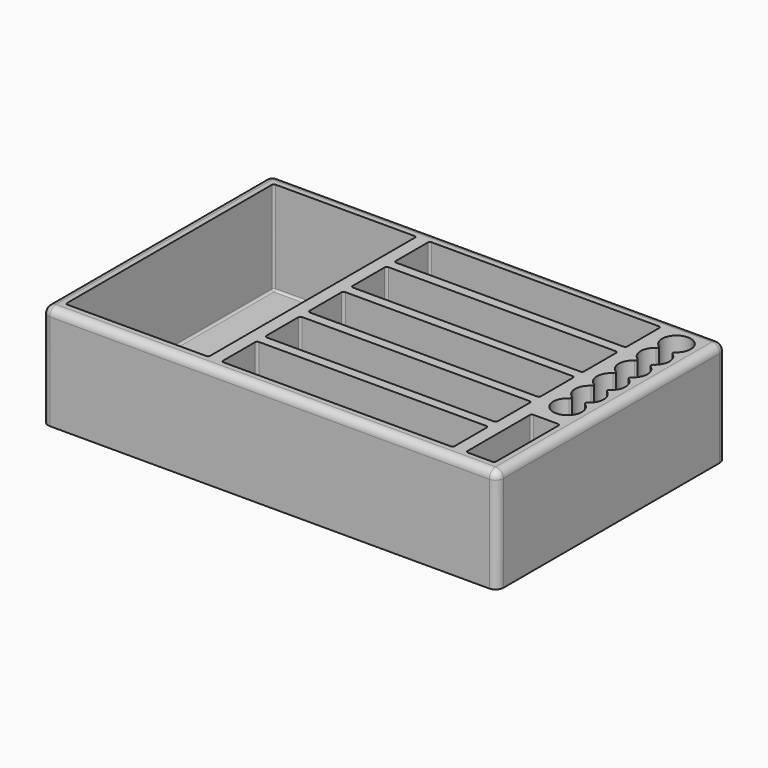
from build123d import *

# Parameters (mm, degrees)
F0_W     = 175
F0_H     = 110
F1_DEPTH = 40
F2_W     = 55
F2_H     = 100
F2_W_2   = 89
F2_H_2   = 17
F2_W_3   = 11
F2_H_3   = 31.5
F3_DEPTH = 36
F4_R     = 0.8068048306
F5_R     = 3


# Not quite as in the source:
# - a feature names something its author has since deleted; it is built from what else it names


with BuildPart() as f1:
    # F0 (on Top) → F1 (new body)
    with BuildSketch(Plane.XY):
        Rectangle(F0_W, F0_H)
    extrude(amount=F1_DEPTH)

    # F2 (on face) → F3 (cut)
    with BuildSketch(Plane.XY.offset(40)):
        with Locations((-55, 0)):
            Rectangle(F2_W, F2_H)
        with Locations((22, 41.5)):
            Rectangle(F2_W_2, F2_H_2)
        with Locations((22, 20.75)):
            Rectangle(F2_W_2, F2_H_2)
        with BuildLine():
            ThreePointArc((78.6393596311, 28.75), (81.4309410948, 30.7416628452), (82.5, 34))
            ThreePointArc((82.5, 34), (81.5093705676, 37.1489009327), (78.8943356059, 39.163476795))
            ThreePointArc((78.8943356059, 39.163476795), (77, 38.8269535899), (75.1056643941, 39.163476795))
            ThreePointArc((75.1056643941, 39.163476795), (71.5016479517, 33.8653717964), (75.3606403689, 28.75))
            ThreePointArc((75.3606403689, 28.75), (77, 29), (78.6393596311, 28.75))
        make_face()
        with BuildLine():
            ThreePointArc((75.1056643941, 39.163476795), (77, 38.8269535899), (78.8943356059, 39.163476795))
            ThreePointArc((78.8943356059, 39.163476795), (77, 39.5), (75.1056643941, 39.163476795))
        make_face()
        with BuildLine():
            ThreePointArc((75.1056643941, 39.163476795), (77, 39.5), (78.8943356059, 39.163476795))
            ThreePointArc((78.8943356059, 39.163476795), (81.5093705676, 41.1780526573), (82.5, 44.3269535899))
            ThreePointArc((82.5, 44.3269535899), (73.8510990673, 48.8363241576), (75.1056643941, 39.163476795))
        make_face()
        with BuildLine():
            ThreePointArc((82.5, 23.5), (81.4309410948, 26.7583371548), (78.6393596311, 28.75))
            ThreePointArc((78.6393596311, 28.75), (77, 28.5), (75.3606403689, 28.75))
            ThreePointArc((75.3606403689, 28.75), (71.5, 23.5), (75.3606403689, 18.25))
            ThreePointArc((75.3606403689, 18.25), (77, 18.5), (78.6393596311, 18.25))
            ThreePointArc((78.6393596311, 18.25), (81.4309410948, 20.2416628452), (82.5, 23.5))
        make_face()
        with BuildLine():
            ThreePointArc((75.3606403689, 28.75), (77, 28.5), (78.6393596311, 28.75))
            ThreePointArc((78.6393596311, 28.75), (77, 29), (75.3606403689, 28.75))
        make_face()
        with BuildLine():
            ThreePointArc((78.6393596311, 18.25), (77, 18.5), (75.3606403689, 18.25))
            ThreePointArc((75.3606403689, 18.25), (77, 18), (78.6393596311, 18.25))
        make_face()
        with BuildLine():
            ThreePointArc((78.6393596311, 18.25), (77, 18), (75.3606403689, 18.25))
            ThreePointArc((75.3606403689, 18.25), (71.5, 13), (75.3606403689, 7.75))
            ThreePointArc((75.3606403689, 7.75), (77, 8), (78.6393596311, 7.75))
            ThreePointArc((78.6393596311, 7.75), (81.4309410948, 9.7416628452), (82.5, 13))
            ThreePointArc((82.5, 13), (81.4309410948, 16.2583371548), (78.6393596311, 18.25))
        make_face()
        with BuildLine():
            ThreePointArc((78.6393596311, 7.75), (77, 8), (75.3606403689, 7.75))
            ThreePointArc((75.3606403689, 7.75), (77, 7.5), (78.6393596311, 7.75))
        make_face()
        with BuildLine():
            ThreePointArc((78.6393596311, 7.75), (77, 7.5), (75.3606403689, 7.75))
            ThreePointArc((75.3606403689, 7.75), (71.5, 2.5), (75.3606403689, -2.75))
            ThreePointArc((75.3606403689, -2.75), (77, -2.5), (78.6393596311, -2.75))
            ThreePointArc((78.6393596311, -2.75), (81.4309410948, -0.7583371548), (82.5, 2.5))
            ThreePointArc((82.5, 2.5), (81.4309410948, 5.7583371548), (78.6393596311, 7.75))
        make_face()
        with BuildLine():
            ThreePointArc((78.6393596311, -2.75), (77, -2.5), (75.3606403689, -2.75))
            ThreePointArc((75.3606403689, -2.75), (77, -3), (78.6393596311, -2.75))
        make_face()
        with BuildLine():
            ThreePointArc((78.6393596311, -2.75), (77, -3), (75.3606403689, -2.75))
            ThreePointArc((75.3606403689, -2.75), (73.7416628452, -12.4309410948), (82.5, -8))
            ThreePointArc((82.5, -8), (81.4309410948, -4.7416628452), (78.6393596311, -2.75))
        make_face()
        with Locations((22, 0)):
            Rectangle(F2_W_2, F2_H_2)
        with Locations((22, -20.75)):
            Rectangle(F2_W_2, F2_H_2)
        with Locations((22, -41.5)):
            Rectangle(F2_W_2, F2_H_2)
        with Locations((77, -34.25)):
            Rectangle(F2_W_3, F2_H_3)
    extrude(amount=-F3_DEPTH, mode=Mode.SUBTRACT)

    # F4
    f4_edges = [f1.edges().sort_by_distance(p)[0] for p in [
        (75.36064, 28.75, 22),
        (75.36064, 18.25, 22),
        (75.36064, 7.75, 22),
        (75.36064, -2.75, 22),
        (78.63936, -2.75, 22),
        (78.63936, 7.75, 22),
        (78.63936, 18.25, 22),
        (78.63936, 28.75, 22),
        (66.5, 50, 22),
        (22, 50, 4),
        (66.5, 41.5, 4),
        (22, 33, 4),
        (-22.5, 41.5, 4),
        (-22.5, 50, 22),
        (-22.5, 33, 22),
        (66.5, 33, 22),
        (66.5, 29.25, 22),
        (22, 29.25, 4),
        (66.5, 20.75, 4),
        (22, 12.25, 4),
        (66.5, 12.25, 22),
        (-22.5, 29.25, 22),
        (-22.5, 20.75, 4),
        (-22.5, 12.25, 22),
        (66.5, 8.5, 22),
        (22, 8.5, 4),
        (66.5, 0, 4),
        (22, -8.5, 4),
        (66.5, -8.5, 22),
        (-22.5, -8.5, 22),
        (-22.5, 8.5, 22),
        (-22.5, 0, 4),
        (66.5, -12.25, 22),
        (66.5, -29.25, 22),
        (66.5, -20.75, 4),
        (22, -29.25, 4),
        (22, -12.25, 4),
        (-22.5, -12.25, 22),
        (-22.5, -20.75, 4),
        (-22.5, -29.25, 22),
        (-22.5, -50, 22),
        (22, -50, 4),
        (-22.5, -41.5, 4),
        (-22.5, -33, 22),
        (22, -33, 4),
        (66.5, -33, 22),
        (66.5, -41.5, 4),
        (66.5, -50, 22),
        (-27.5, 0, 4),
        (-27.5, -50, 22),
        (-55, -50, 4),
        (-27.5, 50, 22),
        (-55, 50, 4),
        (-82.5, 50, 22),
        (-82.5, 0, 4),
        (-82.5, -50, 22),
        (71.5, -18.5, 22),
        (77, -18.5, 4),
        (71.5, -34.25, 4),
        (71.5, -50, 22),
        (77, -50, 4),
        (82.5, -50, 22),
        (82.5, -34.25, 4),
        (82.5, -18.5, 22),
        (78.894336, 39.163477, 22),
        (75.105664, 39.163477, 22),
    ]]
    fillet(f4_edges, radius=F4_R)

    # F5
    f5_edges = [f1.edges().sort_by_distance(p)[0] for p in [
        (-87.5, 0, 40),
        (0, -55, 40),
        (0, 55, 40),
        (87.5, 0, 40),
        (-87.5, -55, 20),
        (-87.5, 55, 20),
        (87.5, 55, 20),
        (87.5, -55, 20),
    ]]
    fillet(f5_edges, radius=F5_R)


solid = f1.part
